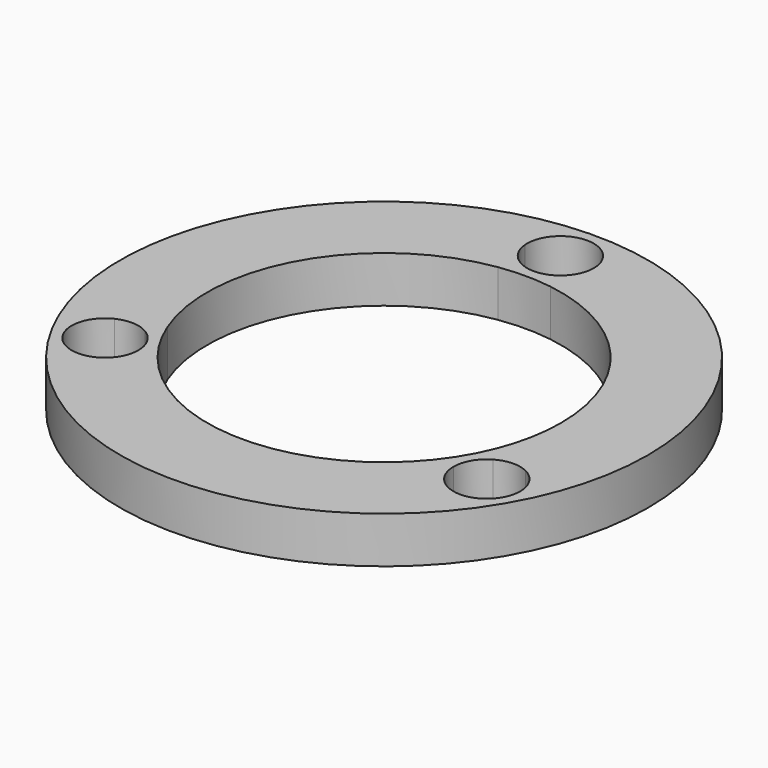
from build123d import *

# Parameters (mm, degrees)
F0_R     = 45.5
F1_DEPTH = 8


with BuildPart() as f1:
    # F0 (on Top) → F1 (new body)
    with BuildSketch(Plane.XY):
        Circle(F0_R)
        with BuildLine():
            ThreePointArc((5.7335195457, 37.5649671053), (28.825975636, 24.7601116442), (38, 0))
            ThreePointArc((38, 0), (37.3440830117, -7.0298978664), (35.3989755783, -13.817109973))
            ThreePointArc((35.3989755783, -13.817109973), (37.7762057759, -15.9385509026), (38.6589653438, -19))
            ThreePointArc((38.6589653438, -19), (35.5933946557, -24.0849129068), (29.6654560327, -23.7478571323))
            ThreePointArc((29.6654560327, -23.7478571323), (0, -38), (-29.6654560327, -23.7478571323))
            ThreePointArc((-29.6654560327, -23.7478571323), (-37.8886114156, -21.875), (-35.3989755783, -13.817109973))
            ThreePointArc((-35.3989755783, -13.817109973), (-32.9089653438, 19), (-5.7335195457, 37.5649671053))
            ThreePointArc((-5.7335195457, 37.5649671053), (-0.2176724746, 43.7458784092), (5.75, 38))
            ThreePointArc((5.75, 38), (5.7458784092, 37.7823275254), (5.7335195457, 37.5649671053))
        make_face(mode=Mode.SUBTRACT)
        with BuildLine():
            ThreePointArc((35.3989755783, -13.817109973), (37.3440830117, -7.0298978664), (38, 0))
            ThreePointArc((38, 0), (28.825975636, 24.7601116442), (5.7335195457, 37.5649671053))
            ThreePointArc((5.7335195457, 37.5649671053), (4.8672404321, 34.9385509026), (2.875, 33.0203539282))
            Line((2.875, 33.0203539282), (4.5250023815, 30.1624659709))
            ThreePointArc((4.5250023815, 30.1624659709), (23.1112804993, 19.9027313121), (30.5, 0))
            ThreePointArc((30.5, 0), (29.9663216824, -5.6806306713), (28.3839629623, -11.1624659709))
            Line((28.3839629623, -11.1624659709), (30.0339653438, -14.0203539282))
            ThreePointArc((30.0339653438, -14.0203539282), (32.6912928692, -13.2541215908), (35.3989755783, -13.817109973))
        make_face()
        with BuildLine():
            ThreePointArc((-2.875, 33.0203539282), (-4.8672404321, 34.9385509026), (-5.7335195457, 37.5649671053))
            ThreePointArc((-5.7335195457, 37.5649671053), (-32.9089653438, 19), (-35.3989755783, -13.817109973))
            ThreePointArc((-35.3989755783, -13.817109973), (-32.6912928692, -13.2541215908), (-30.0339653438, -14.0203539282))
            Line((-30.0339653438, -14.0203539282), (-28.3839629623, -11.1624659709))
            ThreePointArc((-28.3839629623, -11.1624659709), (-26.4137748154, 15.25), (-4.5250023815, 30.1624659709))
            Line((-4.5250023815, 30.1624659709), (-2.875, 33.0203539282))
        make_face()
        with BuildLine():
            ThreePointArc((-29.6654560327, -23.7478571323), (0, -38), (29.6654560327, -23.7478571323))
            ThreePointArc((29.6654560327, -23.7478571323), (27.824052437, -21.6844293119), (27.1589653438, -19))
            Line((27.1589653438, -19), (23.8589605809, -19))
            ThreePointArc((23.8589605809, -19), (0, -30.5), (-23.8589605809, -19))
            Line((-23.8589605809, -19), (-27.1589653438, -19))
            ThreePointArc((-27.1589653438, -19), (-27.824052437, -21.6844293119), (-29.6654560327, -23.7478571323))
        make_face()
        with BuildLine():
            Line((4.5250023815, 30.1624659709), (2.875, 33.0203539282))
            ThreePointArc((2.875, 33.0203539282), (0, 32.25), (-2.875, 33.0203539282))
            Line((-2.875, 33.0203539282), (-4.5250023815, 30.1624659709))
            ThreePointArc((-4.5250023815, 30.1624659709), (0, 30.5), (4.5250023815, 30.1624659709))
        make_face()
        with BuildLine():
            ThreePointArc((27.1589653438, -19), (27.929319272, -16.125), (30.0339653438, -14.0203539282))
            Line((30.0339653438, -14.0203539282), (28.3839629623, -11.1624659709))
            ThreePointArc((28.3839629623, -11.1624659709), (26.4137748154, -15.25), (23.8589605809, -19))
            Line((23.8589605809, -19), (27.1589653438, -19))
        make_face()
        with BuildLine():
            Line((-28.3839629623, -11.1624659709), (-30.0339653438, -14.0203539282))
            ThreePointArc((-30.0339653438, -14.0203539282), (-27.929319272, -16.125), (-27.1589653438, -19))
            Line((-27.1589653438, -19), (-23.8589605809, -19))
            ThreePointArc((-23.8589605809, -19), (-26.4137748154, -15.25), (-28.3839629623, -11.1624659709))
        make_face()
    extrude(amount=F1_DEPTH)


solid = f1.part
